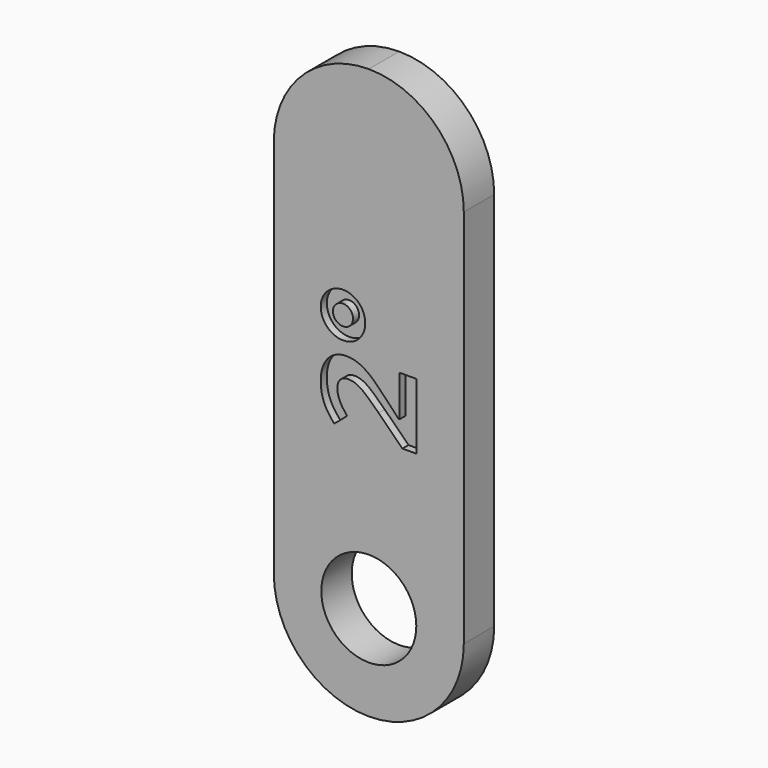
from build123d import *

# Parameters (mm, degrees)
F0_W         = 12.7
F0_H         = 38.1
F0_R         = 3.175
F1_DEPTH     = 2.54
F2_R         = 6.34999
F3_TEXT_SIZE = 8.8194444444
F4_DEPTH     = 0.508


# Not quite as in the source:
# - a fillet or chamfer is up to 0.001 mm smaller than in the source, because OpenCascade refuses the exact size
# - Text() gives the source's letters only with a copy of the font that has no kerning and outlines rounded to 1/6400 em; it was checked with that copy


with BuildPart() as f1:
    # F0 (on Front) → F1 (new body)
    with BuildSketch(Plane.XZ):
        with Locations((6.35, 19.05)):
            Rectangle(F0_W, F0_H)
        with Locations((6.35, 6.35)):
            Circle(F0_R, mode=Mode.SUBTRACT)
    extrude(amount=F1_DEPTH)

    # F2 (radius 6.35 in the source; OpenCascade refuses exactly that, so slightly less here)
    f2_edges = [f1.edges().sort_by_distance(p)[0] for p in [
        (12.7, -1.27, 0),
        (0, -1.27, 0),
        (12.7, -1.27, 38.1),
        (0, -1.27, 38.1),
    ]]
    fillet(f2_edges, radius=F2_R)

    # F3 (on face) → F4 (cut)
    with BuildSketch(Plane.XZ.offset(2.54)):
        with Locations(Location((9.525, 16.1464735243), (0, 0, 90))):
            Text('2°', F3_TEXT_SIZE, font='Open Sans', font_style=FontStyle.BOLD, text_align=(TextAlign.LEFT, TextAlign.BOTTOM))
    extrude(amount=-F4_DEPTH, mode=Mode.SUBTRACT)


solid = f1.part
